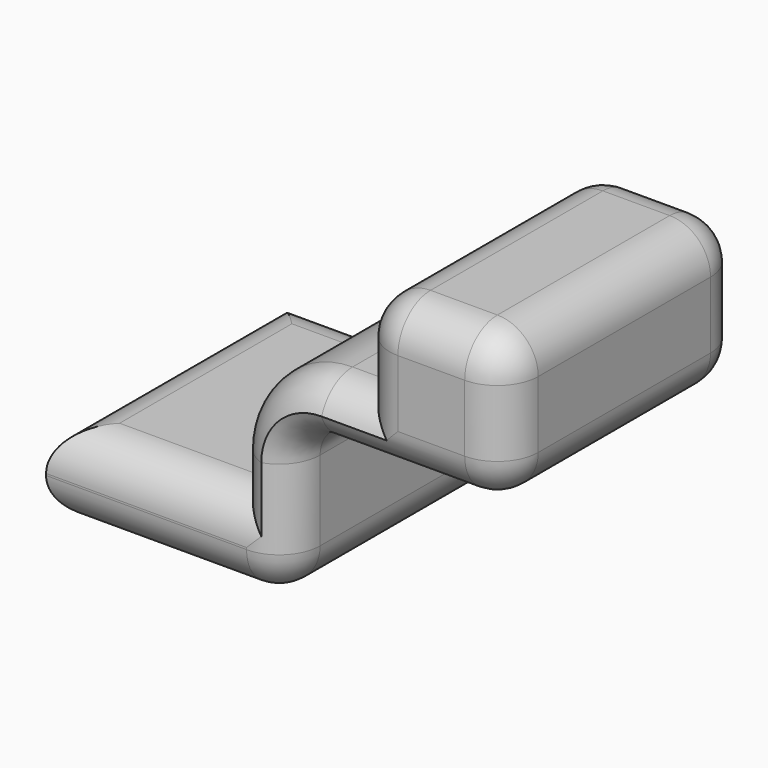
from build123d import *

# Parameters (mm, degrees)
F1_DEPTH      = 101.6
F2_T1_DEPTH   = 22.86
F2_T3_DEPTH   = 17.78
F2_T5_DEPTH   = 73.66
F2_T7_DEPTH   = 22.86
F2_T9_DEPTH   = 49.53
F2_T11_DEPTH  = 12.7
F2_T13_DEPTH  = 98.425
F2_T15_DEPTH  = 171.45
F2_T17_DEPTH  = 103.505
F2_T19_DEPTH  = 12.7
F2_T21_DEPTH  = 27.305
F2_S25_W      = 13.97
F2_S25_H      = 13.97
F2_T26_DEPTH  = 13.97
F2_S31_W      = 13.97
F2_S31_H      = 13.97
F2_T32_DEPTH  = 13.97
F2_S37_W      = 13.97
F2_S37_H      = 13.97
F2_T38_DEPTH  = 13.97
F2_S43_W      = 13.97
F2_S43_H      = 13.97
F2_T44_DEPTH  = 13.97
F2_S49_W      = 13.97
F2_S49_H      = 13.97
F2_T50_DEPTH  = 13.97
F2_S55_W      = 13.97
F2_S55_H      = 13.97
F2_T56_DEPTH  = 13.97
F2_S61_W      = 13.97
F2_S61_H      = 13.97
F2_T62_DEPTH  = 13.97
F2_S67_W      = 13.97
F2_S67_H      = 13.97
F2_T68_DEPTH  = 13.97
F2_T72_ANGLE  = 90
F2_T74_ANGLE  = 90
F2_T76_ANGLE  = 90
F2_T78_ANGLE  = 90
F2_T83_DEPTH  = 52.705
F2_T87_DEPTH  = 47.625
F2_T94_DEPTH  = 47.625
F2_T98_DEPTH  = 52.705
F2_T105_DEPTH = 47.625
F2_T109_DEPTH = 133.35
F2_T116_DEPTH = 133.35
F2_T120_DEPTH = 47.625


# Not quite as in the source:
# - a fillet or chamfer that OpenCascade refuses, or shapes differently, is made with other operations: its cross-section is extruded or revolved along the edge and cut away or added


with BuildPart() as f1:
    # F0 (on Front) → F1 (new body)
    with BuildSketch(Plane.XZ):
        with BuildLine():
            Line((-41.275, -14.2875), (41.275, -14.2875))
            Line((41.275, -14.2875), (41.275, 14.2875))
            Line((41.275, 14.2875), (41.275, 26.9875))
            ThreePointArc((41.275, 26.9875), (44.5297758941, 34.8452241059), (52.3875, 38.1))
            Line((52.3875, 38.1), (65.0875, 38.1))
            Line((65.0875, 38.1), (115.8875, 38.1))
            Line((115.8875, 38.1), (115.8875, 88.9))
            Line((115.8875, 88.9), (65.0875, 88.9))
            Line((65.0875, 88.9), (65.0875, 57.15))
            Line((65.0875, 57.15), (52.3875, 57.15))
            ThreePointArc((52.3875, 57.15), (31.0593917125, 48.3156082875), (22.225, 26.9875))
            Line((22.225, 26.9875), (22.225, 14.2875))
            Line((22.225, 14.2875), (-41.275, 14.2875))
            Line((-41.275, 14.2875), (-41.275, -14.2875))
        make_face()
    extrude(amount=F1_DEPTH)

    # F2: fillet of radius 13.97 on 20 edges, made by hand

    # F2_s2 → F2_t1 (cut)
    with BuildSketch(Plane.YZ.offset(79.0575)):
        with BuildLine():
            ThreePointArc((-101.6, 74.93), (-97.5082817332, 84.8082817332), (-87.63, 88.9))
            Line((-87.63, 88.9), (-101.6, 88.9))
            Line((-101.6, 88.9), (-101.6, 74.93))
        make_face()
        with BuildLine():
            ThreePointArc((-13.97, 88.9), (-4.0917182668, 84.8082817332), (0, 74.93))
            Line((0, 74.93), (0, 88.9))
            Line((0, 88.9), (-13.97, 88.9))
        make_face()
    extrude(amount=F2_T1_DEPTH, mode=Mode.SUBTRACT)

    # F2_s4 → F2_t3 (cut)
    with BuildSketch(Plane.XY.offset(57.15)):
        with BuildLine():
            ThreePointArc((79.0575, -101.6), (69.1792182668, -97.5082817332), (65.0875, -87.63))
            Line((65.0875, -87.63), (65.0875, -101.6))
            Line((65.0875, -101.6), (79.0575, -101.6))
        make_face()
        with BuildLine():
            ThreePointArc((65.0875, -13.97), (69.1792182668, -4.0917182668), (79.0575, 0))
            Line((79.0575, 0), (65.0875, 0))
            Line((65.0875, 0), (65.0875, -13.97))
        make_face()
    extrude(amount=F2_T3_DEPTH, mode=Mode.SUBTRACT)

    # F2_s6 → F2_t5 (cut)
    with BuildSketch(Plane.XZ.offset(13.97)):
        with BuildLine():
            ThreePointArc((101.9175, 88.9), (111.7957817332, 84.8082817332), (115.8875, 74.93))
            Line((115.8875, 74.93), (115.8875, 88.9))
            Line((115.8875, 88.9), (101.9175, 88.9))
        make_face()
        with BuildLine():
            ThreePointArc((65.0875, 74.93), (69.1792182668, 84.8082817332), (79.0575, 88.9))
            Line((79.0575, 88.9), (65.0875, 88.9))
            Line((65.0875, 88.9), (65.0875, 74.93))
        make_face()
        with BuildLine():
            ThreePointArc((115.8875, 52.07), (111.7957817332, 42.1917182668), (101.9175, 38.1))
            Line((101.9175, 38.1), (115.8875, 38.1))
            Line((115.8875, 38.1), (115.8875, 52.07))
        make_face()
        with BuildLine():
            ThreePointArc((27.305, -14.2875), (37.1832817332, -10.1957817332), (41.275, -0.3175))
            Line((41.275, -0.3175), (41.275, -14.2875))
            Line((41.275, -14.2875), (27.305, -14.2875))
        make_face()
    extrude(amount=F2_T5_DEPTH, mode=Mode.SUBTRACT)

    # F2_s8 → F2_t7 (cut)
    with BuildSketch(Plane.XY.offset(52.07)):
        with BuildLine():
            ThreePointArc((101.9175, -101.6), (111.7957817332, -97.5082817332), (115.8875, -87.63))
            Line((115.8875, -87.63), (115.8875, -101.6))
            Line((115.8875, -101.6), (101.9175, -101.6))
        make_face()
        with BuildLine():
            ThreePointArc((115.8875, -13.97), (111.7957817332, -4.0917182668), (101.9175, 0))
            Line((101.9175, 0), (115.8875, 0))
            Line((115.8875, 0), (115.8875, -13.97))
        make_face()
    extrude(amount=F2_T7_DEPTH, mode=Mode.SUBTRACT)

    # F2_s10 → F2_t9 (cut)
    with BuildSketch(Plane.YZ.offset(52.3875)):
        with BuildLine():
            ThreePointArc((-101.6, 52.07), (-97.5082817332, 42.1917182668), (-87.63, 38.1))
            Line((-87.63, 38.1), (-101.6, 38.1))
            Line((-101.6, 38.1), (-101.6, 52.07))
        make_face()
        with BuildLine():
            ThreePointArc((-13.97, 38.1), (-4.0917182668, 42.1917182668), (0, 52.07))
            Line((0, 52.07), (0, 38.1))
            Line((0, 38.1), (-13.97, 38.1))
        make_face()
    extrude(amount=F2_T9_DEPTH, mode=Mode.SUBTRACT)

    # F2_s12 → F2_t11 (cut)
    with BuildSketch(Plane.XY.offset(14.2875)):
        with BuildLine():
            ThreePointArc((36.195, -101.6), (26.3167182668, -97.5082817332), (22.225, -87.63))
            Line((22.225, -87.63), (22.225, -101.6))
            Line((22.225, -101.6), (36.195, -101.6))
        make_face()
        with BuildLine():
            ThreePointArc((22.225, -13.97), (26.3167182668, -4.0917182668), (36.195, 0))
            Line((36.195, 0), (22.225, 0))
            Line((22.225, 0), (22.225, -13.97))
        make_face()
    extrude(amount=F2_T11_DEPTH, mode=Mode.SUBTRACT)

    # F2_s14 → F2_t13 (cut)
    with BuildSketch(Plane.YZ.offset(-76.2)):
        with BuildLine():
            ThreePointArc((-101.6, 0.3175), (-97.5082817332, 10.1957817332), (-87.63, 14.2875))
            Line((-87.63, 14.2875), (-101.6, 14.2875))
            Line((-101.6, 14.2875), (-101.6, 0.3175))
        make_face()
        with BuildLine():
            ThreePointArc((-13.97, 14.2875), (-4.0917182668, 10.1957817332), (0, 0.3175))
            Line((0, 0.3175), (0, 14.2875))
            Line((0, 14.2875), (-13.97, 14.2875))
        make_face()
    extrude(amount=F2_T13_DEPTH, mode=Mode.SUBTRACT)

    # F2_s16 → F2_t15 (cut)
    with BuildSketch(Plane.XZ.offset(-34.925)):
        with BuildLine():
            ThreePointArc((-27.305, 14.2875), (-37.1832817332, 10.1957817332), (-41.275, 0.3175))
            Line((-41.275, 0.3175), (-41.275, 14.2875))
            Line((-41.275, 14.2875), (-27.305, 14.2875))
        make_face()
        with BuildLine():
            ThreePointArc((-27.305, -14.2875), (-37.1832817332, -10.1957817332), (-41.275, -0.3175))
            Line((-41.275, -0.3175), (-41.275, -14.2875))
            Line((-41.275, -14.2875), (-27.305, -14.2875))
        make_face()
    extrude(amount=F2_T15_DEPTH, mode=Mode.SUBTRACT)

    # F2_s18 → F2_t17 (cut)
    with BuildSketch(Plane.YZ.offset(-76.2)):
        with BuildLine():
            ThreePointArc((-13.97, -14.2875), (-4.0917182668, -10.1957817332), (0, -0.3175))
            Line((0, -0.3175), (0, -14.2875))
            Line((0, -14.2875), (-13.97, -14.2875))
        make_face()
        with BuildLine():
            ThreePointArc((-87.63, -14.2875), (-97.5082817332, -10.1957817332), (-101.6, -0.3175))
            Line((-101.6, -0.3175), (-101.6, -14.2875))
            Line((-101.6, -14.2875), (-87.63, -14.2875))
        make_face()
    extrude(amount=F2_T17_DEPTH, mode=Mode.SUBTRACT)

    # F2_s20 → F2_t19 (cut)
    with BuildSketch(Plane.YZ.offset(52.3875)):
        with BuildLine():
            ThreePointArc((-13.97, 57.15), (-4.0917182668, 53.0582817332), (0, 43.18))
            Line((0, 43.18), (0, 57.15))
            Line((0, 57.15), (-13.97, 57.15))
        make_face()
        with BuildLine():
            ThreePointArc((-101.6, 43.18), (-97.5082817332, 53.0582817332), (-87.63, 57.15))
            Line((-87.63, 57.15), (-101.6, 57.15))
            Line((-101.6, 57.15), (-101.6, 43.18))
        make_face()
    extrude(amount=F2_T19_DEPTH, mode=Mode.SUBTRACT)

    # F2_s22 → F2_t21 (cut)
    with BuildSketch(Plane.XY.offset(-0.3175)):
        with BuildLine():
            ThreePointArc((27.305, 0), (37.1832817332, -4.0917182668), (41.275, -13.97))
            Line((41.275, -13.97), (41.275, 0))
            Line((41.275, 0), (27.305, 0))
        make_face()
        with BuildLine():
            ThreePointArc((27.305, -101.6), (37.1832817332, -97.5082817332), (41.275, -87.63))
            Line((41.275, -87.63), (41.275, -101.6))
            Line((41.275, -101.6), (27.305, -101.6))
        make_face()
    extrude(amount=F2_T21_DEPTH, mode=Mode.SUBTRACT)


with BuildPart() as f2_tool24:
    # F2_s25 → F2_t26 (new body)
    with BuildSketch(Plane.YZ.offset(101.9175)):
        with Locations((-94.615, 81.915)):
            Rectangle(F2_S25_W, F2_S25_H)
    extrude(amount=F2_T26_DEPTH)

    # F2_s27 → F2_t28 (revolve, cut)
    with BuildSketch(Plane(origin=(101.9175, -87.63, 74.93), x_dir=(0, 0.7071067812, -0.7071067812), z_dir=(0, -0.7071067812, -0.7071067812))):
        with BuildLine():
            ThreePointArc((0, -13.97), (13.97, 0), (0, 13.97))
            Line((0, 13.97), (0, -13.97))
        make_face()
    revolve(axis=Axis((101.9175, -87.63, 74.93), (1, 0, 0)), mode=Mode.SUBTRACT)


with BuildPart() as f1_1:
    add(f1.part)

    # F2_t23: cut F2_tool24
    add(f2_tool24.part, mode=Mode.SUBTRACT)


with BuildPart() as f2_tool30:
    # F2_s31 → F2_t32 (new body)
    with BuildSketch(Plane.XZ.offset(87.63)):
        with Locations((72.0725, 81.915)):
            Rectangle(F2_S31_W, F2_S31_H)
    extrude(amount=F2_T32_DEPTH)

    # F2_s33 → F2_t34 (revolve, cut)
    with BuildSketch(Plane(origin=(79.0575, -87.63, 74.93), x_dir=(0.7071067812, 0, -0.7071067812), z_dir=(-0.7071067812, 0, -0.7071067812))):
        with BuildLine():
            ThreePointArc((0, -13.97), (13.97, 0), (0, 13.97))
            Line((0, 13.97), (0, -13.97))
        make_face()
    revolve(axis=Axis((79.0575, -87.63, 74.93), (0, -1, 0)), mode=Mode.SUBTRACT)


with BuildPart() as f1_2:
    add(f1_1.part)

    # F2_t29: cut F2_tool30
    add(f2_tool30.part, mode=Mode.SUBTRACT)


with BuildPart() as f2_tool36:
    # F2_s37 → F2_t38 (new body)
    with BuildSketch(Plane.YZ.offset(101.9175)):
        with Locations((-6.985, 81.915)):
            Rectangle(F2_S37_W, F2_S37_H)
    extrude(amount=F2_T38_DEPTH)

    # F2_s39 → F2_t40 (revolve, cut)
    with BuildSketch(Plane(origin=(101.9175, -13.97, 74.93), x_dir=(0, -0.7071067812, -0.7071067812), z_dir=(0, -0.7071067812, 0.7071067812))):
        with BuildLine():
            ThreePointArc((0, -13.97), (13.97, 0), (0, 13.97))
            Line((0, 13.97), (0, -13.97))
        make_face()
    revolve(axis=Axis((101.9175, -13.97, 74.93), (1, 0, 0)), mode=Mode.SUBTRACT)


with BuildPart() as f1_3:
    add(f1_2.part)

    # F2_t35: cut F2_tool36
    add(f2_tool36.part, mode=Mode.SUBTRACT)


with BuildPart() as f2_tool42:
    # F2_s43 → F2_t44 (new body)
    with BuildSketch(Plane.XZ.offset(13.97)):
        with Locations((72.0725, 81.915)):
            Rectangle(F2_S43_W, F2_S43_H)
    extrude(amount=-F2_T44_DEPTH)

    # F2_s45 → F2_t46 (revolve, cut)
    with BuildSketch(Plane(origin=(79.0575, -13.97, 74.93), x_dir=(0.7071067812, 0, -0.7071067812), z_dir=(0.7071067812, 0, 0.7071067812))):
        with BuildLine():
            ThreePointArc((0, -13.97), (13.97, 0), (0, 13.97))
            Line((0, 13.97), (0, -13.97))
        make_face()
    revolve(axis=Axis((79.0575, -13.97, 74.93), (0, 1, 0)), mode=Mode.SUBTRACT)


with BuildPart() as f1_4:
    add(f1_3.part)

    # F2_t41: cut F2_tool42
    add(f2_tool42.part, mode=Mode.SUBTRACT)


with BuildPart() as f2_tool48:
    # F2_s49 → F2_t50 (new body)
    with BuildSketch(Plane.YZ.offset(101.9175)):
        with Locations((-94.615, 45.085)):
            Rectangle(F2_S49_W, F2_S49_H)
    extrude(amount=F2_T50_DEPTH)

    # F2_s51 → F2_t52 (revolve, cut)
    with BuildSketch(Plane(origin=(101.9175, -87.63, 52.07), x_dir=(0, 0.7071067812, 0.7071067812), z_dir=(0, 0.7071067812, -0.7071067812))):
        with BuildLine():
            ThreePointArc((0, -13.97), (13.97, 0), (0, 13.97))
            Line((0, 13.97), (0, -13.97))
        make_face()
    revolve(axis=Axis((101.9175, -87.63, 52.07), (1, 0, 0)), mode=Mode.SUBTRACT)


with BuildPart() as f1_5:
    add(f1_4.part)

    # F2_t47: cut F2_tool48
    add(f2_tool48.part, mode=Mode.SUBTRACT)


with BuildPart() as f2_tool54:
    # F2_s55 → F2_t56 (new body)
    with BuildSketch(Plane.YZ.offset(101.9175)):
        with Locations((-6.985, 45.085)):
            Rectangle(F2_S55_W, F2_S55_H)
    extrude(amount=F2_T56_DEPTH)

    # F2_s57 → F2_t58 (revolve, cut)
    with BuildSketch(Plane(origin=(101.9175, -13.97, 52.07), x_dir=(0, -0.7071067812, 0.7071067812), z_dir=(0, 0.7071067812, 0.7071067812))):
        with BuildLine():
            ThreePointArc((0, -13.97), (13.97, 0), (0, 13.97))
            Line((0, 13.97), (0, -13.97))
        make_face()
    revolve(axis=Axis((101.9175, -13.97, 52.07), (1, 0, 0)), mode=Mode.SUBTRACT)


with BuildPart() as f1_6:
    add(f1_5.part)

    # F2_t53: cut F2_tool54
    add(f2_tool54.part, mode=Mode.SUBTRACT)


with BuildPart() as f2_tool60:
    # F2_s61 → F2_t62 (new body)
    with BuildSketch(Plane.XY.offset(-0.3175)):
        with Locations((34.29, -6.985)):
            Rectangle(F2_S61_W, F2_S61_H)
    extrude(amount=-F2_T62_DEPTH)

    # F2_s63 → F2_t64 (revolve, cut)
    with BuildSketch(Plane(origin=(27.305, -13.97, -0.3175), x_dir=(-0.7071067812, -0.7071067812, 0), z_dir=(0.7071067812, -0.7071067812, 0))):
        with BuildLine():
            ThreePointArc((0, -13.97), (13.97, 0), (0, 13.97))
            Line((0, 13.97), (0, -13.97))
        make_face()
    revolve(axis=Axis((27.305, -13.97, -0.3175), (0, 0, -1)), mode=Mode.SUBTRACT)


with BuildPart() as f1_7:
    add(f1_6.part)

    # F2_t59: cut F2_tool60
    add(f2_tool60.part, mode=Mode.SUBTRACT)


with BuildPart() as f2_tool66:
    # F2_s67 → F2_t68 (new body)
    with BuildSketch(Plane.XY.offset(-0.3175)):
        with Locations((34.29, -94.615)):
            Rectangle(F2_S67_W, F2_S67_H)
    extrude(amount=-F2_T68_DEPTH)

    # F2_s69 → F2_t70 (revolve, cut)
    with BuildSketch(Plane(origin=(27.305, -87.63, -0.3175), x_dir=(-0.7071067812, 0.7071067812, 0), z_dir=(-0.7071067812, -0.7071067812, 0))):
        with BuildLine():
            ThreePointArc((0, -13.97), (13.97, 0), (0, 13.97))
            Line((0, 13.97), (0, -13.97))
        make_face()
    revolve(axis=Axis((27.305, -87.63, -0.3175), (0, 0, -1)), mode=Mode.SUBTRACT)


with BuildPart() as f1_8:
    add(f1_7.part)

    # F2_t65: cut F2_tool66
    add(f2_tool66.part, mode=Mode.SUBTRACT)

    # F2_s71 → F2_t72 (revolve, cut)
    with BuildSketch(Plane.YZ.offset(52.3875)):
        with BuildLine():
            ThreePointArc((-13.97, 57.15), (-4.0917182668, 53.0582817332), (0, 43.18))
            Line((0, 43.18), (0, 57.15))
            Line((0, 57.15), (-13.97, 57.15))
        make_face()
    revolve(axis=Axis((52.3875, 0, 26.9875), (0, -1, 0)), revolution_arc=F2_T72_ANGLE, mode=Mode.SUBTRACT)

    # F2_s73 → F2_t74 (revolve, cut)
    with BuildSketch(Plane.YZ.offset(52.3875)):
        with BuildLine():
            ThreePointArc((-101.6, 43.18), (-97.5082817332, 53.0582817332), (-87.63, 57.15))
            Line((-87.63, 57.15), (-101.6, 57.15))
            Line((-101.6, 57.15), (-101.6, 43.18))
        make_face()
    revolve(axis=Axis((52.3875, -101.6, 26.9875), (0, -1, 0)), revolution_arc=F2_T74_ANGLE, mode=Mode.SUBTRACT)

    # F2_s75 → F2_t76 (revolve, cut)
    with BuildSketch(Plane.XY.offset(26.9875)):
        with BuildLine():
            ThreePointArc((41.275, -13.97), (37.1832817332, -4.0917182668), (27.305, 0))
            Line((27.305, 0), (41.275, 0))
            Line((41.275, 0), (41.275, -13.97))
        make_face()
    revolve(axis=Axis((52.3875, 0, 26.9875), (0, 1, 0)), revolution_arc=F2_T76_ANGLE, mode=Mode.SUBTRACT)

    # F2_s77 → F2_t78 (revolve, cut)
    with BuildSketch(Plane.XY.offset(26.9875)):
        with BuildLine():
            ThreePointArc((27.305, -101.6), (37.1832817332, -97.5082817332), (41.275, -87.63))
            Line((41.275, -87.63), (41.275, -101.6))
            Line((41.275, -101.6), (27.305, -101.6))
        make_face()
    revolve(axis=Axis((52.3875, -101.6, 26.9875), (0, 1, 0)), revolution_arc=F2_T78_ANGLE, mode=Mode.SUBTRACT)


with BuildPart() as f2_tool81:
    # F2_s82 → F2_t83 (new body)
    with BuildSketch(Plane.XY.offset(74.93)):
        with BuildLine():
            ThreePointArc((79.0575, -101.6), (69.1792182668, -97.5082817332), (65.0875, -87.63))
            Line((65.0875, -87.63), (65.0875, -101.6))
            Line((65.0875, -101.6), (79.0575, -101.6))
        make_face()
    extrude(amount=-F2_T83_DEPTH)

    split(bisect_by=Plane.XY.offset(57.15), keep=Keep.BOTTOM)


with BuildPart() as f2_tool85:
    # F2_s86 → F2_t87 (new body)
    with BuildSketch(Plane.YZ.offset(100.0125)):
        with BuildLine():
            ThreePointArc((-101.6, 43.18), (-97.5082817332, 53.0582817332), (-87.63, 57.15))
            Line((-87.63, 57.15), (-101.6, 57.15))
            Line((-101.6, 57.15), (-101.6, 43.18))
        make_face()
    extrude(amount=-F2_T87_DEPTH)

    split(bisect_by=Plane.YZ.offset(65.0875), keep=Keep.TOP)


with BuildPart() as f2_tool81_1:
    add(f2_tool81.part)

    # F2_t89: intersect F2_tool85
    add(f2_tool85.part, mode=Mode.INTERSECT)


with BuildPart() as f1_9:
    add(f1_8.part)

    # F2_t79: cut F2_tool81
    add(f2_tool81_1.part, mode=Mode.SUBTRACT)


with BuildPart() as f2_tool92:
    # F2_s93 → F2_t94 (new body)
    with BuildSketch(Plane.YZ.offset(100.0125)):
        with BuildLine():
            ThreePointArc((-13.97, 57.15), (-4.0917182668, 53.0582817332), (0, 43.18))
            Line((0, 43.18), (0, 57.15))
            Line((0, 57.15), (-13.97, 57.15))
        make_face()
    extrude(amount=-F2_T94_DEPTH)

    split(bisect_by=Plane.YZ.offset(65.0875), keep=Keep.TOP)


with BuildPart() as f2_tool96:
    # F2_s97 → F2_t98 (new body)
    with BuildSketch(Plane.XY.offset(74.93)):
        with BuildLine():
            ThreePointArc((65.0875, -13.97), (69.1792182668, -4.0917182668), (79.0575, 0))
            Line((79.0575, 0), (65.0875, 0))
            Line((65.0875, 0), (65.0875, -13.97))
        make_face()
    extrude(amount=-F2_T98_DEPTH)

    split(bisect_by=Plane.XY.offset(57.15), keep=Keep.BOTTOM)


with BuildPart() as f2_tool92_1:
    add(f2_tool92.part)

    # F2_t100: intersect F2_tool96
    add(f2_tool96.part, mode=Mode.INTERSECT)


with BuildPart() as f1_10:
    add(f1_9.part)

    # F2_t90: cut F2_tool92
    add(f2_tool92_1.part, mode=Mode.SUBTRACT)


with BuildPart() as f2_tool103:
    # F2_s104 → F2_t105 (new body)
    with BuildSketch(Plane.XY.offset(26.9875)):
        with BuildLine():
            ThreePointArc((36.195, -101.6), (26.3167182668, -97.5082817332), (22.225, -87.63))
            Line((22.225, -87.63), (22.225, -101.6))
            Line((22.225, -101.6), (36.195, -101.6))
        make_face()
    extrude(amount=-F2_T105_DEPTH)

    split(bisect_by=Plane.XY.offset(14.2875), keep=Keep.BOTTOM)


with BuildPart() as f2_tool107:
    # F2_s108 → F2_t109 (new body)
    with BuildSketch(Plane.YZ.offset(57.15)):
        with BuildLine():
            ThreePointArc((-101.6, 0.3175), (-97.5082817332, 10.1957817332), (-87.63, 14.2875))
            Line((-87.63, 14.2875), (-101.6, 14.2875))
            Line((-101.6, 14.2875), (-101.6, 0.3175))
        make_face()
    extrude(amount=-F2_T109_DEPTH)

    split(bisect_by=Plane.YZ.offset(22.225), keep=Keep.TOP)


with BuildPart() as f2_tool103_1:
    add(f2_tool103.part)

    # F2_t111: intersect F2_tool107
    add(f2_tool107.part, mode=Mode.INTERSECT)


with BuildPart() as f1_11:
    add(f1_10.part)

    # F2_t101: cut F2_tool103
    add(f2_tool103_1.part, mode=Mode.SUBTRACT)


with BuildPart() as f2_tool114:
    # F2_s115 → F2_t116 (new body)
    with BuildSketch(Plane.YZ.offset(57.15)):
        with BuildLine():
            ThreePointArc((-13.97, 14.2875), (-4.0917182668, 10.1957817332), (0, 0.3175))
            Line((0, 0.3175), (0, 14.2875))
            Line((0, 14.2875), (-13.97, 14.2875))
        make_face()
    extrude(amount=-F2_T116_DEPTH)

    split(bisect_by=Plane.YZ.offset(22.225), keep=Keep.TOP)


with BuildPart() as f2_tool118:
    # F2_s119 → F2_t120 (new body)
    with BuildSketch(Plane.XY.offset(26.9875)):
        with BuildLine():
            ThreePointArc((22.225, -13.97), (26.3167182668, -4.0917182668), (36.195, 0))
            Line((36.195, 0), (22.225, 0))
            Line((22.225, 0), (22.225, -13.97))
        make_face()
    extrude(amount=-F2_T120_DEPTH)

    split(bisect_by=Plane.XY.offset(14.2875), keep=Keep.BOTTOM)


with BuildPart() as f2_tool114_1:
    add(f2_tool114.part)

    # F2_t122: intersect F2_tool118
    add(f2_tool118.part, mode=Mode.INTERSECT)


with BuildPart() as f1_12:
    add(f1_11.part)

    # F2_t112: cut F2_tool114
    add(f2_tool114_1.part, mode=Mode.SUBTRACT)


solid = f1_12.part
